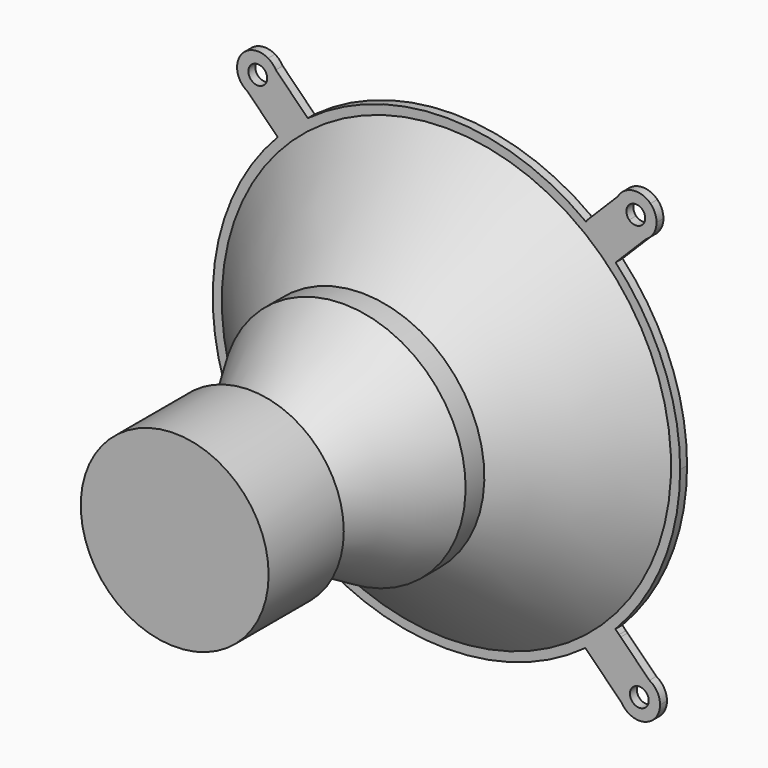
from build123d import *

# Parameters (mm, degrees)
F0_R         = 63.5
F1_DEPTH     = 63.5
F4_T         = -2.54
F6_START     = 180.594
F5_R         = 106.1598946296
F6_DEPTH     = 34.544
F7_T2_ANGLE  = 90
F7_T4_ANGLE  = 270
F8_TEXT_SIZE = 75.7205197352
F9_DEPTH     = 0.3556
F11_START    = -166.116
F10_R        = 148.8542413229
F11_DEPTH    = 5.842


# Not quite as in the source:
# - a fillet or chamfer that OpenCascade refuses, or shapes differently, is made with other operations: its cross-section is extruded or revolved along the edge and cut away or added
# - Text() gives the source's letters only with a copy of the font that has no kerning and outlines rounded to 1/6400 em; it was checked with that copy


with BuildPart() as f1:
    # F0 (on Front) → F1 (new body)
    with BuildSketch(Plane.XZ):
        Circle(F0_R)
    extrude(amount=F1_DEPTH)

    # F2 (on Right) → F3 (revolve)
    with BuildSketch(Plane.YZ):
        Polygon((79.1459254743, 82.5531298544), (0, 36.9198411355), (0, 0), (166.6873318047, 0), (166.6873318047, 152.4), (94.9778789028, 82.5531298544), align=None)
    revolve(axis=Axis((0, 83.3436659024, 0), (0, -1, 0)))

    # F4
    f4_openings = [f1.faces().sort_by_distance(p)[0] for p in [
        (0, 166.687332, 0),
    ]]
    offset(amount=F4_T, openings=f4_openings, kind=Kind.INTERSECTION)

    # F5 (on face) → F6 (join)
    with BuildSketch(Plane(origin=(0, -60.96, 0), x_dir=(-1, 0, 0), z_dir=(0, 1, 0)).offset(F6_START)):
        Circle(F5_R)
    extrude(amount=F6_DEPTH)

    # F7: fillet of radius 55.1889220358 on 1 edges, made by hand

    # F7_s1 → F7_t2 (revolve, cut)
    with BuildSketch(Plane.XY):
        with BuildLine():
            ThreePointArc((-106.1598946296, 122.8544694732), (-85.7977898508, 145.6951929108), (-56.3978588633, 154.178))
            Line((-56.3978588633, 154.178), (-106.1598946296, 154.178))
            Line((-106.1598946296, 154.178), (-106.1598946296, 122.8544694732))
        make_face()
    revolve(axis=Axis((0, 154.178, 0), (0, 1, 0)), revolution_arc=F7_T2_ANGLE, mode=Mode.SUBTRACT)

    # F7_s3 → F7_t4 (revolve, cut)
    with BuildSketch(Plane.YZ):
        with BuildLine():
            ThreePointArc((122.8544694732, 106.1598946296), (145.6951929108, 85.7977898508), (154.178, 56.3978588633))
            Line((154.178, 56.3978588633), (154.178, 106.1598946296))
            Line((154.178, 106.1598946296), (122.8544694732, 106.1598946296))
        make_face()
    revolve(axis=Axis((0, 154.178, 0), (0, 1, 0)), revolution_arc=F7_T4_ANGLE, mode=Mode.SUBTRACT)

    # F8 (on face) → F9 (join)
    with BuildSketch(Plane(origin=(0, 154.178, 0), x_dir=(-1, 0, 0), z_dir=(0, 1, 0))):
        with Locations((-48.26, -27.6255248298)):
            Text('EV', F8_TEXT_SIZE, font='Open Sans', font_style=FontStyle.BOLD, text_align=(TextAlign.LEFT, TextAlign.BOTTOM))
    extrude(amount=F9_DEPTH)

    # F10 (on Front) → F11 (join)
    with BuildSketch(Plane.XZ.offset(F11_START)):
        with BuildLine():
            ThreePointArc((114.2095973396, -109.1769762205), (146.6430356051, -58.8155113013), (157.9982413229, 0))
            ThreePointArc((157.9982413229, 0), (146.68356491, 58.7143597973), (114.3600841188, 109.0193350808))
            ThreePointArc((114.3600841188, 109.0193350808), (109.5970253669, 113.8065740273), (104.6337496526, 118.3859058113))
            ThreePointArc((104.6337496526, 118.3859058113), (99.5676290294, 122.6773471778), (94.325685516, 126.7521570351))
            ThreePointArc((94.325685516, 126.7521570351), (0.3606877801, 157.9978296226), (-93.7459891555, 127.1814993557))
            ThreePointArc((-93.7459891555, 127.1814993557), (-99.1227321445, 123.0371010441), (-104.3164831167, 118.6655620274))
            ThreePointArc((-104.3164831167, 118.6655620274), (-109.2920536928, 114.099479669), (-114.0679599542, 109.3249503682))
            ThreePointArc((-114.0679599542, 109.3249503682), (-157.9979687689, -0.2934723165), (-113.6610444075, -109.7479441507))
            ThreePointArc((-113.6610444075, -109.7479441507), (-108.9742497945, -114.4030469124), (-104.0969685206, -118.8581734923))
            ThreePointArc((-104.0969685206, -118.8581734923), (-99.0089814808, -123.1286556706), (-93.7459891555, -127.1814993557))
            ThreePointArc((-93.7459891555, -127.1814993557), (0.1005887073, -157.9982093032), (93.9078519267, -127.0620305506))
            ThreePointArc((93.9078519267, -127.0620305506), (99.3655406795, -122.8410907904), (104.6337496526, -118.3859058113))
            ThreePointArc((104.6337496526, -118.3859058113), (109.5185086035, -113.8821343951), (114.2095973396, -109.1769762205))
        make_face()
        Circle(F10_R, mode=Mode.SUBTRACT)
        with BuildLine():
            ThreePointArc((104.6337496526, 118.3859058113), (109.5970253669, 113.8065740273), (114.3600841188, 109.0193350808))
            Line((114.3600841188, 109.0193350808), (134.9541818099, 129.672383262))
            ThreePointArc((134.9541818099, 129.672383262), (126.1645776628, 127.962151386), (118.1353232036, 131.9261275416))
            Line((118.1353232036, 131.9261275416), (104.6337496526, 118.3859058113))
        make_face()
        with BuildLine():
            Line((116.7149224195, -111.6873530388), (114.2095973396, -109.1769762205))
            ThreePointArc((114.2095973396, -109.1769762205), (109.5185086035, -113.8821343951), (104.6337496526, -118.3859058113))
            Line((104.6337496526, -118.3859058113), (120.6580494517, -134.4102056105))
            ThreePointArc((120.6580494517, -134.4102056105), (128.5741185501, -130.5814494889), (137.2123289639, -132.2260905608))
            Line((137.2123289639, -132.2260905608), (117.7991926935, -112.7738096357))
            Line((117.7991926935, -112.7738096357), (116.7149224195, -111.6873530388))
        make_face()
        with BuildLine():
            ThreePointArc((94.325685516, 126.7521570351), (99.5676290294, 122.6773471778), (104.6337496526, 118.3859058113))
            Line((104.6337496526, 118.3859058113), (118.1353232036, 131.9261275416))
            ThreePointArc((118.1353232036, 131.9261275416), (114.1484124407, 139.9440185799), (115.8335131474, 148.738475342))
            Line((115.8335131474, 148.738475342), (95.2394154563, 128.0854271607))
            Line((95.2394154563, 128.0854271607), (94.325685516, 126.7521570351))
        make_face()
        with BuildLine():
            ThreePointArc((118.1353232036, 131.9261275416), (126.1645776628, 127.962151386), (134.9541818099, 129.672383262))
            Line((134.9541818099, 129.672383262), (140.215966534, 134.9492298156))
            ThreePointArc((140.215966534, 134.9492298156), (141.5692858283, 138.2791498809), (142.0305183387, 141.8438525788))
            ThreePointArc((142.0305183387, 141.8438525788), (140.9605585281, 147.212877278), (137.9141564777, 151.761577616))
            Line((137.9141564777, 151.761577616), (132.5084460234, 146.3403933455))
            ThreePointArc((132.5084460234, 146.3403933455), (133.8896368671, 144.278084053), (134.3747398407, 141.8438525788))
            ThreePointArc((134.3747398407, 141.8438525788), (130.4589713149, 135.9789555524), (123.541033658, 137.3473118121))
            Line((123.541033658, 137.3473118121), (118.1353232036, 131.9261275416))
        make_face()
        with BuildLine():
            Line((140.215966534, 134.9492298156), (134.9541818099, 129.672383262))
            ThreePointArc((134.9541818099, 129.672383262), (137.9424648779, 131.9544359417), (140.215966534, 134.9492298156))
        make_face()
        with BuildLine():
            Line((120.6580494517, -134.4102056105), (104.6337496526, -118.3859058113))
            ThreePointArc((104.6337496526, -118.3859058113), (99.3655406795, -122.8410907904), (93.9078519267, -127.0620305506))
            Line((93.9078519267, -127.0620305506), (97.6203049086, -130.781969324))
            Line((97.6203049086, -130.781969324), (99.0955262982, -132.2601653505))
            Line((99.0955262982, -132.2601653505), (118.2909277908, -151.4942724573))
            ThreePointArc((118.2909277908, -151.4942724573), (116.5328753118, -142.5446571246), (120.6580494517, -134.4102056105))
        make_face()
        with BuildLine():
            ThreePointArc((115.8335131474, 148.738475342), (114.1484124407, 139.9440185799), (118.1353232036, 131.9261275416))
            Line((118.1353232036, 131.9261275416), (123.541033658, 137.3473118121))
            ThreePointArc((123.541033658, 137.3473118121), (123.5281990739, 146.3275587615), (132.5084460234, 146.3403933455))
            Line((132.5084460234, 146.3403933455), (137.9141564777, 151.761577616))
            ThreePointArc((137.9141564777, 151.761577616), (129.8849020185, 155.7255537716), (121.0952978714, 154.0153218956))
            Line((121.0952978714, 154.0153218956), (115.8335131474, 148.738475342))
        make_face()
        with BuildLine():
            ThreePointArc((137.2123289639, -132.2260905608), (128.5741185501, -130.5814494889), (120.6580494517, -134.4102056105))
            ThreePointArc((120.6580494517, -134.4102056105), (116.5328753118, -142.5446571246), (118.2909277908, -151.4942724573))
            Line((118.2909277908, -151.4942724573), (123.3543497974, -156.5679043498))
            ThreePointArc((123.3543497974, -156.5679043498), (137.3845244006, -156.6103571822), (144.4118953414, -144.4668955958))
            ThreePointArc((144.4118953414, -144.4668955958), (142.4785675206, -137.3663487167), (137.2123289639, -132.2260905608))
        make_face()
        with BuildLine():
            ThreePointArc((135.0479038253, -148.800059984), (125.9159887829, -148.9570236564), (126.0729524552, -139.825108614))
            ThreePointArc((126.0729524552, -139.825108614), (132.9366213519, -138.6428895062), (136.7561168434, -144.4668955958))
            ThreePointArc((136.7561168434, -144.4668955958), (136.3136479409, -146.7957528977), (135.0479038253, -148.800059984))
        make_face(mode=Mode.SUBTRACT)
        with BuildLine():
            ThreePointArc((-104.3164831167, 118.6655620274), (-99.1227321445, 123.0371010441), (-93.7459891555, 127.1814993557))
            Line((-93.7459891555, 127.1814993557), (-115.3162415471, 148.9007442222))
            ThreePointArc((-115.3162415471, 148.9007442222), (-113.9731999814, 145.5817498869), (-113.5155500756, 142.0306879883))
            ThreePointArc((-113.5155500756, 142.0306879883), (-114.5909189646, 136.6486499828), (-117.6518911536, 132.0930818955))
            Line((-117.6518911536, 132.0930818955), (-104.3164831167, 118.6655620274))
        make_face()
        with BuildLine():
            ThreePointArc((121.0952978714, 154.0153218956), (118.1070148035, 151.7332692158), (115.8335131474, 148.738475342))
            Line((115.8335131474, 148.738475342), (121.0952978714, 154.0153218956))
        make_face()
        with BuildLine():
            Line((-116.7659431854, -150.2014533857), (-93.7459891555, -127.1814993557))
            ThreePointArc((-93.7459891555, -127.1814993557), (-99.0089814808, -123.1286556706), (-104.0969685206, -118.8581734923))
            Line((-104.0969685206, -118.8581734923), (-119.93776155, -134.6989665217))
            ThreePointArc((-119.93776155, -134.6989665217), (-116.7799462733, -139.2989939719), (-115.6685458737, -144.7667941708))
            ThreePointArc((-115.6685458737, -144.7667941708), (-115.9456361793, -147.5389684818), (-116.7659431854, -150.2014533857))
        make_face()
        with BuildLine():
            Line((123.3543497974, -156.5679043498), (118.2909277908, -151.4942724573))
            ThreePointArc((118.2909277908, -151.4942724573), (120.4925661845, -154.3604967939), (123.3543497974, -156.5679043498))
        make_face()
        with BuildLine():
            ThreePointArc((-114.0679599542, 109.3249503682), (-109.2920536928, 114.099479669), (-104.3164831167, 118.6655620274))
            Line((-104.3164831167, 118.6655620274), (-117.6518911536, 132.0930818955))
            ThreePointArc((-117.6518911536, 132.0930818955), (-125.6890965945, 128.1452749928), (-134.4752326304, 129.8731824548))
            Line((-134.4752326304, 129.8731824548), (-114.0679599542, 109.3249503682))
        make_face()
        with BuildLine():
            ThreePointArc((-113.5155500756, 142.0306879883), (-113.9731999814, 145.5817498869), (-115.3162415471, 148.9007442222))
            Line((-115.3162415471, 148.9007442222), (-120.5674193207, 154.1881935218))
            ThreePointArc((-120.5674193207, 154.1881935218), (-129.3535553567, 155.9161009838), (-137.3907607975, 151.9682940811))
            Line((-137.3907607975, 151.9682940811), (-131.9959735472, 146.5362433492))
            ThreePointArc((-131.9959735472, 146.5362433492), (-125.0811940201, 147.893132533), (-121.1713259756, 142.0306879883))
            ThreePointArc((-121.1713259756, 142.0306879883), (-121.6588814308, 139.5905560328), (-123.0466784039, 137.5251326274))
            Line((-123.0466784039, 137.5251326274), (-117.6518911536, 132.0930818955))
            ThreePointArc((-117.6518911536, 132.0930818955), (-114.5909189646, 136.6486499828), (-113.5155500756, 142.0306879883))
        make_face()
        with BuildLine():
            Line((-120.5674193207, 154.1881935218), (-115.3162415471, 148.9007442222))
            ThreePointArc((-115.3162415471, 148.9007442222), (-117.5837198827, 151.9001228102), (-120.5674193207, 154.1881935218))
        make_face()
        with BuildLine():
            Line((-119.93776155, -134.6989665217), (-104.0969685206, -118.8581734923))
            ThreePointArc((-104.0969685206, -118.8581734923), (-108.9742497945, -114.4030469124), (-113.6610444075, -109.7479441507))
            Line((-113.6610444075, -109.7479441507), (-136.3882138207, -132.4751135639))
            ThreePointArc((-136.3882138207, -132.4751135639), (-127.7980192338, -130.8872679779), (-119.93776155, -134.6989665217))
        make_face()
        with BuildLine():
            ThreePointArc((-136.3882138207, -132.4751135639), (-139.0630755114, -155.159727434), (-116.7659431854, -150.2014533857))
            ThreePointArc((-116.7659431854, -150.2014533857), (-115.9456361793, -147.5389684818), (-115.6685458737, -144.7667941708))
            ThreePointArc((-115.6685458737, -144.7667941708), (-116.7799462733, -139.2989939719), (-119.93776155, -134.6989665217))
            ThreePointArc((-119.93776155, -134.6989665217), (-127.7980192338, -130.8872679779), (-136.3882138207, -132.4751135639))
        make_face()
        with BuildLine():
            ThreePointArc((-134.3270275243, -149.088232496), (-134.1644498342, -140.2766661103), (-125.3528834485, -140.1140884202))
            ThreePointArc((-125.3528834485, -140.1140884202), (-123.8535128366, -142.2289440339), (-123.3243217737, -144.7667941708))
            ThreePointArc((-123.3243217737, -144.7667941708), (-127.3529193437, -150.6772586837), (-134.3270275243, -149.088232496))
        make_face(mode=Mode.SUBTRACT)
        with BuildLine():
            ThreePointArc((-134.4752326304, 129.8731824548), (-125.6890965945, 128.1452749928), (-117.6518911536, 132.0930818955))
            Line((-117.6518911536, 132.0930818955), (-123.0466784039, 137.5251326274))
            ThreePointArc((-123.0466784039, 137.5251326274), (-132.0268813364, 137.5560404167), (-131.9959735472, 146.5362433492))
            Line((-131.9959735472, 146.5362433492), (-137.3907607975, 151.9682940811))
            ThreePointArc((-137.3907607975, 151.9682940811), (-141.3937979346, 143.9584536134), (-139.726410404, 135.1606317544))
            Line((-139.726410404, 135.1606317544), (-134.4752326304, 129.8731824548))
        make_face()
        with BuildLine():
            ThreePointArc((-139.726410404, 135.1606317544), (-137.4589320684, 132.1612531663), (-134.4752326304, 129.8731824548))
            Line((-134.4752326304, 129.8731824548), (-139.726410404, 135.1606317544))
        make_face()
    extrude(amount=-F11_DEPTH)


solid = f1.part
